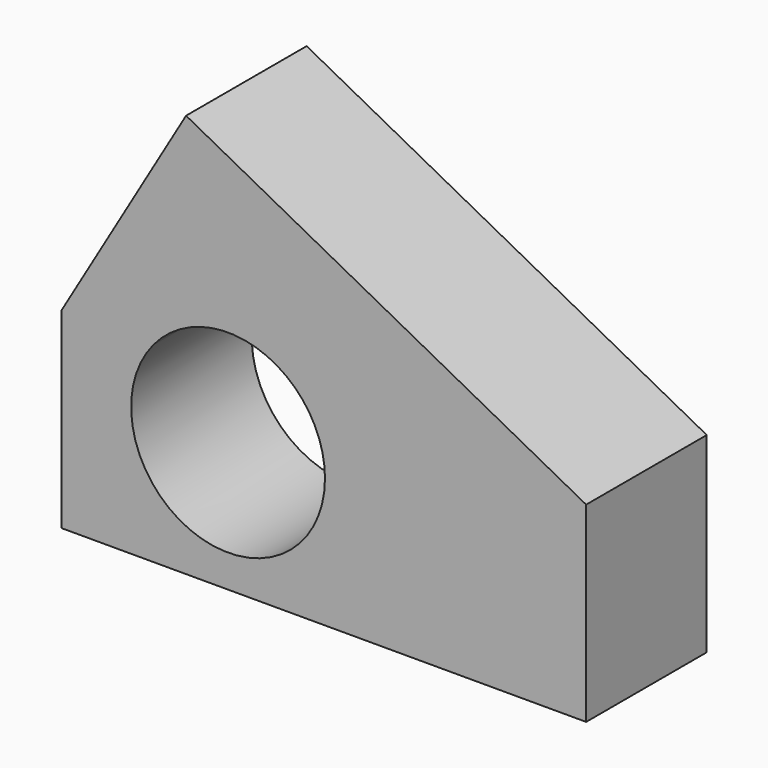
from build123d import *

# Parameters (mm, degrees)
F1_DEPTH = 25.4


# Not quite as in the source:
# - a feature names something its author has since deleted; it is built from what else it names


with BuildPart() as f1:
    # F0 (on Front) → F1 (new body)
    with BuildSketch(Plane.XZ):
        with BuildLine():
            Line((-23.1970027089, 51.8983751535), (-44.2315712571, 16.1199513823))
            Line((-44.2315712571, 16.1199513823), (-28.70137633, 16.1199513823))
            ThreePointArc((-28.70137633, 16.1199513823), (-16.1199513823, 22.0364309456), (-3.5385264346, 16.1199513823))
            Line((-3.5385264346, 16.1199513823), (44.2315712571, 16.1199513823))
            Line((44.2315712571, 16.1199513823), (-23.1970027089, 51.8983751535))
        make_face()
        with BuildLine():
            Line((-28.70137633, 16.1199513823), (-44.2315712571, 16.1199513823))
            Line((-44.2315712571, 16.1199513823), (-44.2315712571, -16.1199513823))
            Line((-44.2315712571, -16.1199513823), (44.2315712571, -16.1199513823))
            Line((44.2315712571, -16.1199513823), (44.2315712571, 16.1199513823))
            Line((44.2315712571, 16.1199513823), (-3.5385264346, 16.1199513823))
            ThreePointArc((-3.5385264346, 16.1199513823), (-0.7516202277, 11.2382926218), (0.215521602, 5.7009579614))
            ThreePointArc((0.215521602, 5.7009579614), (-21.6572860427, -9.6673731932), (-28.70137633, 16.1199513823))
        make_face()
    extrude(amount=F1_DEPTH)


solid = f1.part
